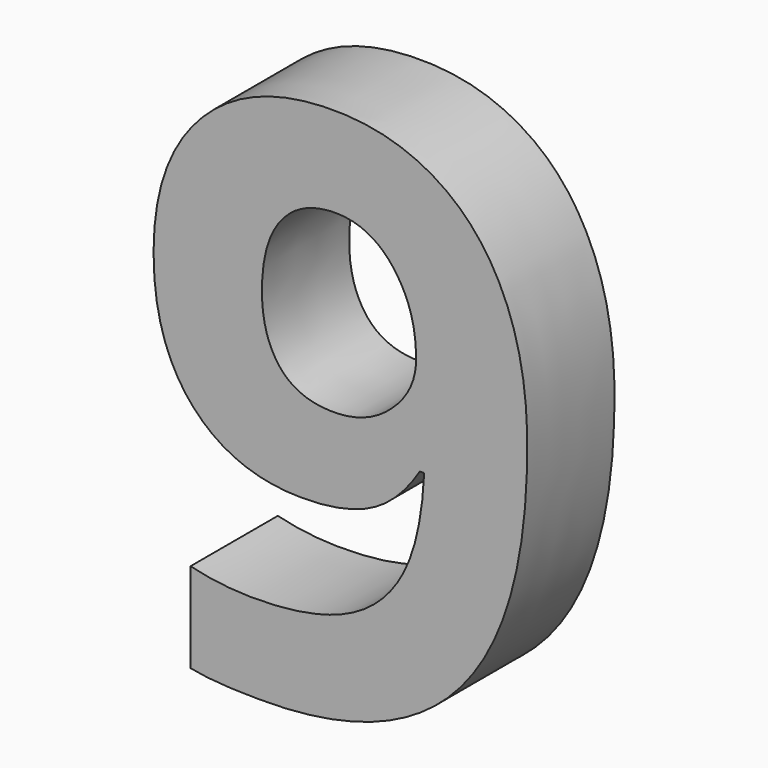
from build123d import *

# Parameters (mm, degrees)
F0_TEXT_SIZE = 34.5463424714
F1_DEPTH     = 5.08


# Not quite as in the source:
# - Text() gives the source's letters only with a copy of the font that has no kerning and outlines rounded to 1/6400 em; it was checked with that copy


with BuildPart() as f1:
    # F0 (on Front) → F1 (new body)
    with BuildSketch(Plane.XZ):
        with Locations((-20.7601926789, 25.1052435488)):
            Text('9', F0_TEXT_SIZE, font='Open Sans', font_style=FontStyle.BOLD, text_align=(TextAlign.LEFT, TextAlign.BOTTOM))
    extrude(amount=F1_DEPTH)


solid = f1.part
